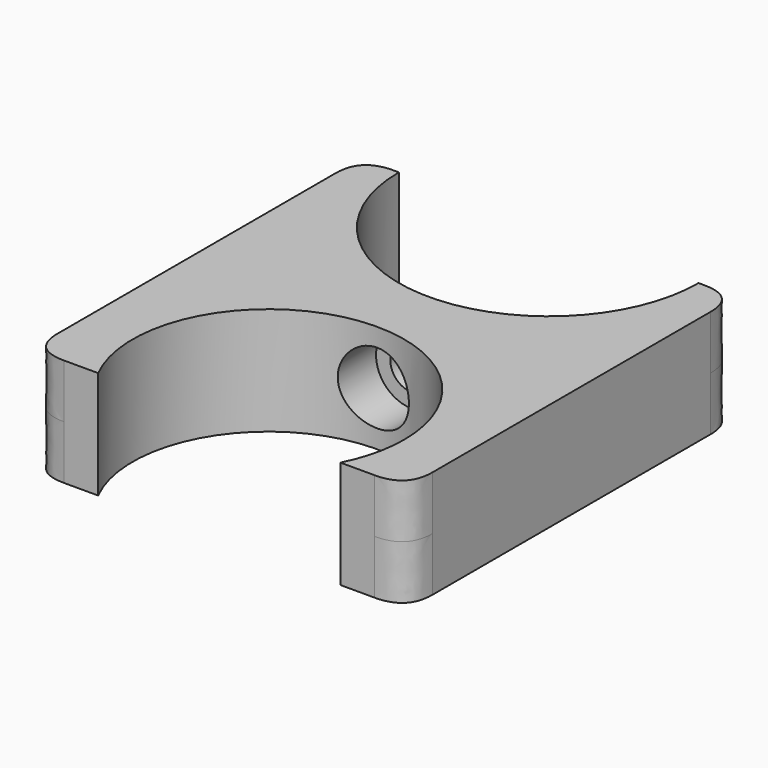
from build123d import *

# Parameters (mm, degrees)
F1_DEPTH      = 6.35
F1_DEPTH_BACK = 6.35
F2_R          = 4.191
F2_R_2        = 2.5019
F3_DEPTH      = 4.064
F3_DEPTH_BACK = 24.258
F4_DEPTH      = 24.258
F5_T1_DEPTH   = 15.875
F5_T3_DEPTH   = 15.875


# Not quite as in the source:
# - a fillet or chamfer that OpenCascade refuses, or shapes differently, is made with other operations: its cross-section is extruded or revolved along the edge and cut away or added
# - a feature names something its author has since deleted; it is built from what else it names


with BuildPart() as f1:
    # F0 (on Top) → F1 (new body, two sides)
    with BuildSketch(Plane.XY) as f1_sk:
        with BuildLine():
            Line((22.098, 24.257), (17.653, 24.257))
            ThreePointArc((17.653, 24.257), (0, 6.604), (-17.653, 24.257))
            Line((-17.653, 24.257), (-22.098, 24.257))
            Line((-22.098, 24.257), (-22.098, -24.257))
            Line((-22.098, -24.257), (-14.2709804499, -24.257))
            ThreePointArc((-14.2709804498, -24.257), (-3.7215436879, -1.454770368), (16.002, -17.018))
            ThreePointArc((16.002, -17.018), (15.563229632, -20.7395436879), (14.2709804499, -24.257))
            Line((14.2709804499, -24.257), (22.098, -24.257))
            Line((22.098, -24.257), (22.098, 24.257))
        make_face()
    extrude(amount=F1_DEPTH)
    extrude(f1_sk.sketch, amount=-F1_DEPTH_BACK)

    # F2 (on Front) → F3 (cut, two sides)
    with BuildSketch(Plane.XZ) as f3_sk:
        Circle(F2_R)
        Circle(F2_R_2, mode=Mode.SUBTRACT)
        Circle(F2_R_2)
    extrude(amount=-F3_DEPTH, mode=Mode.SUBTRACT)
    extrude(f3_sk.sketch, amount=F3_DEPTH_BACK, mode=Mode.SUBTRACT)

    # F2 (on Front) → F4 (cut, through all)
    with BuildSketch(Plane.XZ):
        Circle(F2_R_2)
    extrude(amount=-F4_DEPTH, mode=Mode.SUBTRACT)

    # F5: fillet of radius 3.81 on 8 edges, made by hand

    # F5_s2 → F5_t1 (cut)
    with BuildSketch(Plane.XY):
        with BuildLine():
            add(Edge.make_bspline(
                [(-22.098, -20.447), (-22.098, -24.257), (-18.288, -24.257)],
                knots=[0, 0, 0, 1, 1, 1], degree=2, weights=[1, 1, 1]))
            Line((-18.288, -24.257), (-22.098, -24.257))
            Line((-22.098, -24.257), (-22.098, -20.447))
        make_face()
        with BuildLine():
            add(Edge.make_bspline(
                [(18.288, -24.257), (22.098, -24.257), (22.098, -20.447)],
                knots=[0, 0, 0, 1, 1, 1], degree=2, weights=[1, 1, 1]))
            Line((22.098, -20.447), (22.098, -24.257))
            Line((22.098, -24.257), (18.288, -24.257))
        make_face()
        with BuildLine():
            add(Edge.make_bspline(
                [(-18.288, 24.257), (-22.098, 24.257), (-22.098, 20.447)],
                knots=[0, 0, 0, 1, 1, 1], degree=2, weights=[1, 1, 1]))
            Line((-22.098, 20.447), (-22.098, 24.257))
            Line((-22.098, 24.257), (-18.288, 24.257))
        make_face()
        with BuildLine():
            add(Edge.make_bspline(
                [(22.098, 20.447), (22.098, 24.257), (18.288, 24.257)],
                knots=[0, 0, 0, 1, 1, 1], degree=2, weights=[1, 1, 1]))
            Line((18.288, 24.257), (22.098, 24.257))
            Line((22.098, 24.257), (22.098, 20.447))
        make_face()
    extrude(amount=F5_T1_DEPTH, mode=Mode.SUBTRACT)

    # F5_s4 → F5_t3 (cut)
    with BuildSketch(Plane.XY.offset(-15.875)):
        with BuildLine():
            add(Edge.make_bspline(
                [(-22.098, -20.447), (-22.098, -24.257), (-18.288, -24.257)],
                knots=[0, 0, 0, 1, 1, 1], degree=2, weights=[1, 1, 1]))
            Line((-18.288, -24.257), (-22.098, -24.257))
            Line((-22.098, -24.257), (-22.098, -20.447))
        make_face()
        with BuildLine():
            add(Edge.make_bspline(
                [(18.288, -24.257), (22.098, -24.257), (22.098, -20.447)],
                knots=[0, 0, 0, 1, 1, 1], degree=2, weights=[1, 1, 1]))
            Line((22.098, -20.447), (22.098, -24.257))
            Line((22.098, -24.257), (18.288, -24.257))
        make_face()
        with BuildLine():
            add(Edge.make_bspline(
                [(-18.288, 24.257), (-22.098, 24.257), (-22.098, 20.447)],
                knots=[0, 0, 0, 1, 1, 1], degree=2, weights=[1, 1, 1]))
            Line((-22.098, 20.447), (-22.098, 24.257))
            Line((-22.098, 24.257), (-18.288, 24.257))
        make_face()
        with BuildLine():
            add(Edge.make_bspline(
                [(22.098, 20.447), (22.098, 24.257), (18.288, 24.257)],
                knots=[0, 0, 0, 1, 1, 1], degree=2, weights=[1, 1, 1]))
            Line((18.288, 24.257), (22.098, 24.257))
            Line((22.098, 24.257), (22.098, 20.447))
        make_face()
    extrude(amount=F5_T3_DEPTH, mode=Mode.SUBTRACT)


solid = f1.part
